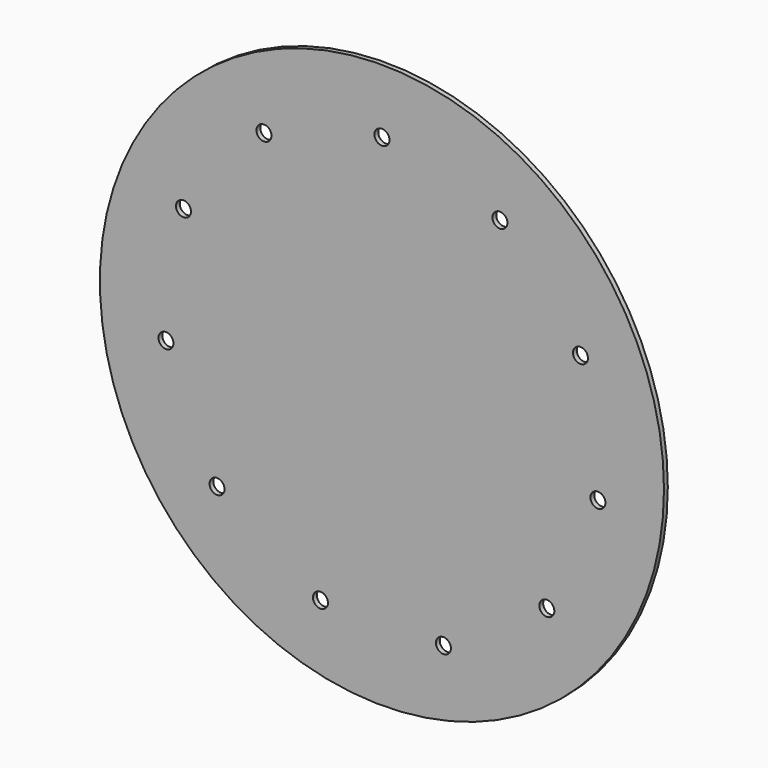
from build123d import *

# Parameters (mm, degrees)
F0_R            = 29.845
F1_DEPTH        = 0.508
F2_D            = 1.5875
F2_COPIES_COUNT = 11


# Not quite as in the source:
# - a pattern or mirror of a feature is missing from the dataset's text; its kind, count and spacing are read off the source's solid


with BuildPart() as f1:
    # F0 (on Front) → F1 (new body)
    with BuildSketch(Plane.XZ):
        Circle(F0_R)
    extrude(amount=F1_DEPTH)

    # F2 (through all)
    with Locations(Plane(origin=(0, 0, 0), x_dir=(1, 0, 0), z_dir=(0, 1, 0))):
        with Locations((0, -23.0886)):
            f2 = Hole(F2_D / 2)

    # F2_copies: F2 ×11 about axis
    f2_copies_axis = Axis((0, 0, 0), (0, 1, 0))
    for i in range(1, F2_COPIES_COUNT):
        add(f2.rotate(f2_copies_axis, i * 360 / F2_COPIES_COUNT), mode=Mode.SUBTRACT)


solid = f1.part
